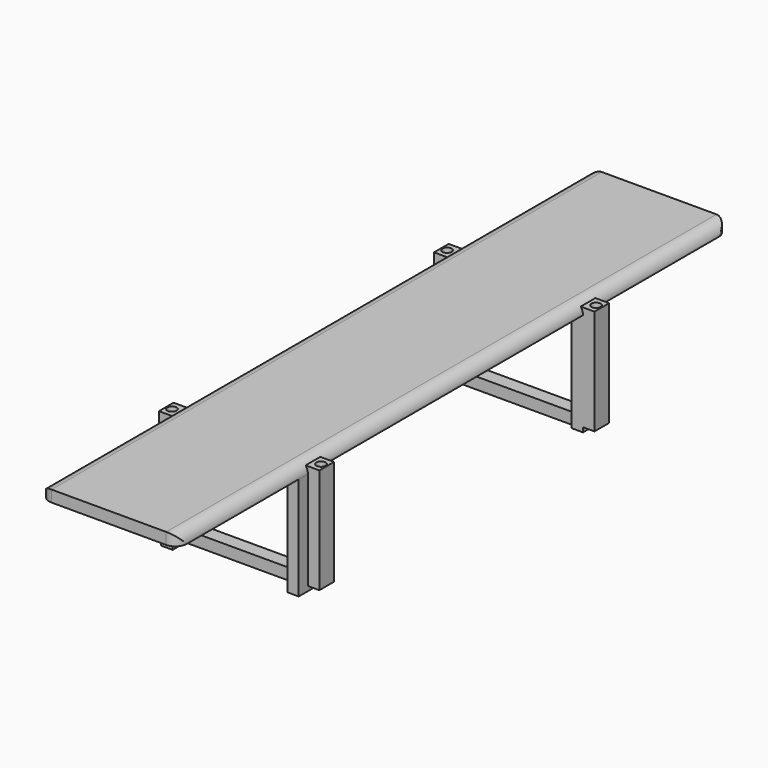
from build123d import *

# Parameters (mm, degrees)
F2_DEPTH      = 300
F3_W          = 8
F3_H          = 46
F4_DEPTH      = 5
F5_W          = 8
F5_H          = 46
F6_DEPTH      = 5
F7_W          = 50
F7_H          = 6
F8_DEPTH      = 5
F9_W          = 66
F9_H          = 45
F10_DEPTH     = 65.001
F11_R         = 2
F12_DEPTH     = 50.001
F13_T1_DEPTH  = 30
F13_T6_DEPTH  = 325
F13_T11_DEPTH = 325
F13_T16_DEPTH = 325
F13_T22_DEPTH = 325
F13_T27_DEPTH = 325
F13_T32_DEPTH = 325
F13_T37_DEPTH = 325
F13_T43_DEPTH = 325


# Not quite as in the source:
# - a fillet or chamfer that OpenCascade refuses, or shapes differently, is made with other operations: its cross-section is extruded or revolved along the edge and cut away or added


with BuildPart() as f2:
    # F1 (on face) → F2 (new body)
    with BuildSketch(Plane.XZ):
        Polygon((0, 0), (5, 0), (5, 45), (55, 45), (55, 0), (60, 0), (60, 50), (0, 50), align=None)
    extrude(amount=F2_DEPTH)

    # F3 (on face) → F4 (join)
    with BuildSketch(Plane.YZ.offset(60)):
        with Locations((-225, 25)):
            Rectangle(F3_W, F3_H)
        with Locations((-75, 25)):
            Rectangle(F3_W, F3_H)
    extrude(amount=F4_DEPTH)

    # F5 (on face) → F6 (join)
    with BuildSketch(Plane(origin=(0, 0, 0), x_dir=(0, -1, 0), z_dir=(-1, 0, 0))):
        with Locations((75, 25)):
            Rectangle(F5_W, F5_H)
        with Locations((225, 25)):
            Rectangle(F5_W, F5_H)
    extrude(amount=F6_DEPTH)

    # F7 (on face) → F8 (join)
    with BuildSketch(Plane(origin=(0, 0, 0), x_dir=(1, 0, 0), z_dir=(0, 0, -1))):
        with Locations((30, 74)):
            Rectangle(F7_W, F7_H)
        with Locations((30, 224)):
            Rectangle(F7_W, F7_H)
    extrude(amount=-F8_DEPTH)

    # F9 (on face) → F10 (cut, through all)
    with BuildSketch(Plane(origin=(0, 0, 0), x_dir=(0, -1, 0), z_dir=(-1, 0, 0))):
        Polygon((221, 45), (79, 45), (79, 2), (79, 0), (221, 0), (221, 2), align=None)
        with Locations((33, 22.5)):
            Rectangle(F9_W, F9_H)
        with Locations((267, 22.5)):
            Rectangle(F9_W, F9_H)
    extrude(amount=-F10_DEPTH, mode=Mode.SUBTRACT)

    # F11 (on Top) → F12 (cut, through all)
    with BuildSketch(Plane.XY):
        with Locations((-2.5, -75)):
            Circle(F11_R)
        with Locations((62.5, -75)):
            Circle(F11_R)
        with Locations((-2.5, -225)):
            Circle(F11_R)
        with Locations((62.5, -225)):
            Circle(F11_R)
    extrude(amount=F12_DEPTH, mode=Mode.SUBTRACT)

    # F13: fillet of radius 5 on 6 edges, made by hand

    # F13_s2 → F13_t1 (cut)
    with BuildSketch(Plane.XY.offset(32.5)):
        with BuildLine():
            ThreePointArc((0, -295), (1.4644660941, -298.5355339059), (5, -300))
            Line((5, -300), (0, -300))
            Line((0, -300), (0, -295))
        make_face()
        with BuildLine():
            ThreePointArc((60, -295), (58.5355339059, -298.5355339059), (55, -300))
            Line((55, -300), (60, -300))
            Line((60, -300), (60, -295))
        make_face()
        with BuildLine():
            ThreePointArc((60, -5), (58.5355339059, -1.4644660941), (55, 0))
            Line((55, 0), (60, 0))
            Line((60, 0), (60, -5))
        make_face()
        with BuildLine():
            ThreePointArc((0, -5), (1.4644660941, -1.4644660941), (5, 0))
            Line((5, 0), (0, 0))
            Line((0, 0), (0, -5))
        make_face()
    extrude(amount=F13_T1_DEPTH, mode=Mode.SUBTRACT)


with BuildPart() as f13_tool4:
    # F13_s5 → F13_t6 (new body)
    with BuildSketch(Plane.XZ.offset(-12.5)):
        with BuildLine():
            ThreePointArc((0, 45), (1.4644660941, 48.5355339059), (5, 50))
            Line((5, 50), (0, 50))
            Line((0, 50), (0, 45))
        make_face()
    extrude(amount=F13_T6_DEPTH)

    split(bisect_by=Plane.XZ.offset(71), keep=Keep.BOTTOM)


with BuildPart() as f2_1:
    add(f2.part)

    # F13_t3: cut F13_tool4
    add(f13_tool4.part, mode=Mode.SUBTRACT)


with BuildPart() as f13_tool9:
    # F13_s10 → F13_t11 (new body)
    with BuildSketch(Plane.XZ.offset(-12.5)):
        with BuildLine():
            ThreePointArc((0, 45), (1.4644660941, 48.5355339059), (5, 50))
            Line((5, 50), (0, 50))
            Line((0, 50), (0, 45))
        make_face()
    extrude(amount=F13_T11_DEPTH)

    split(bisect_by=Plane.XY.offset(48), keep=Keep.TOP)


with BuildPart() as f2_2:
    add(f2_1.part)

    # F13_t8: cut F13_tool9
    add(f13_tool9.part, mode=Mode.SUBTRACT)


with BuildPart() as f13_tool14:
    # F13_s15 → F13_t16 (new body)
    with BuildSketch(Plane.XZ.offset(-12.5)):
        with BuildLine():
            ThreePointArc((0, 45), (1.4644660941, 48.5355339059), (5, 50))
            Line((5, 50), (0, 50))
            Line((0, 50), (0, 45))
        make_face()
    extrude(amount=F13_T16_DEPTH)

    split(bisect_by=Plane.XZ.offset(79), keep=Keep.TOP)

    split(bisect_by=Plane.XZ.offset(221), keep=Keep.BOTTOM)


with BuildPart() as f2_3:
    add(f2_2.part)

    # F13_t13: cut F13_tool14
    add(f13_tool14.part, mode=Mode.SUBTRACT)


with BuildPart() as f13_tool20:
    # F13_s21 → F13_t22 (new body)
    with BuildSketch(Plane.XZ.offset(-12.5)):
        with BuildLine():
            ThreePointArc((0, 45), (1.4644660941, 48.5355339059), (5, 50))
            Line((5, 50), (0, 50))
            Line((0, 50), (0, 45))
        make_face()
    extrude(amount=F13_T22_DEPTH)

    split(bisect_by=Plane.XZ.offset(229), keep=Keep.TOP)


with BuildPart() as f2_4:
    add(f2_3.part)

    # F13_t19: cut F13_tool20
    add(f13_tool20.part, mode=Mode.SUBTRACT)


with BuildPart() as f13_tool25:
    # F13_s26 → F13_t27 (new body)
    with BuildSketch(Plane.XZ.offset(-12.5)):
        with BuildLine():
            ThreePointArc((60, 45), (58.5355339059, 48.5355339059), (55, 50))
            Line((55, 50), (60, 50))
            Line((60, 50), (60, 45))
        make_face()
    extrude(amount=F13_T27_DEPTH)

    split(bisect_by=Plane.XZ.offset(71), keep=Keep.BOTTOM)


with BuildPart() as f2_5:
    add(f2_4.part)

    # F13_t24: cut F13_tool25
    add(f13_tool25.part, mode=Mode.SUBTRACT)


with BuildPart() as f13_tool30:
    # F13_s31 → F13_t32 (new body)
    with BuildSketch(Plane.XZ.offset(-12.5)):
        with BuildLine():
            ThreePointArc((60, 45), (58.5355339059, 48.5355339059), (55, 50))
            Line((55, 50), (60, 50))
            Line((60, 50), (60, 45))
        make_face()
    extrude(amount=F13_T32_DEPTH)

    split(bisect_by=Plane.XY.offset(48), keep=Keep.TOP)


with BuildPart() as f2_6:
    add(f2_5.part)

    # F13_t29: cut F13_tool30
    add(f13_tool30.part, mode=Mode.SUBTRACT)


with BuildPart() as f13_tool35:
    # F13_s36 → F13_t37 (new body)
    with BuildSketch(Plane.XZ.offset(-12.5)):
        with BuildLine():
            ThreePointArc((60, 45), (58.5355339059, 48.5355339059), (55, 50))
            Line((55, 50), (60, 50))
            Line((60, 50), (60, 45))
        make_face()
    extrude(amount=F13_T37_DEPTH)

    split(bisect_by=Plane.XZ.offset(79), keep=Keep.TOP)

    split(bisect_by=Plane.XZ.offset(221), keep=Keep.BOTTOM)


with BuildPart() as f2_7:
    add(f2_6.part)

    # F13_t34: cut F13_tool35
    add(f13_tool35.part, mode=Mode.SUBTRACT)


with BuildPart() as f13_tool41:
    # F13_s42 → F13_t43 (new body)
    with BuildSketch(Plane.XZ.offset(-12.5)):
        with BuildLine():
            ThreePointArc((60, 45), (58.5355339059, 48.5355339059), (55, 50))
            Line((55, 50), (60, 50))
            Line((60, 50), (60, 45))
        make_face()
    extrude(amount=F13_T43_DEPTH)

    split(bisect_by=Plane.XZ.offset(229), keep=Keep.TOP)


with BuildPart() as f2_8:
    add(f2_7.part)

    # F13_t40: cut F13_tool41
    add(f13_tool41.part, mode=Mode.SUBTRACT)


solid = f2_8.part
